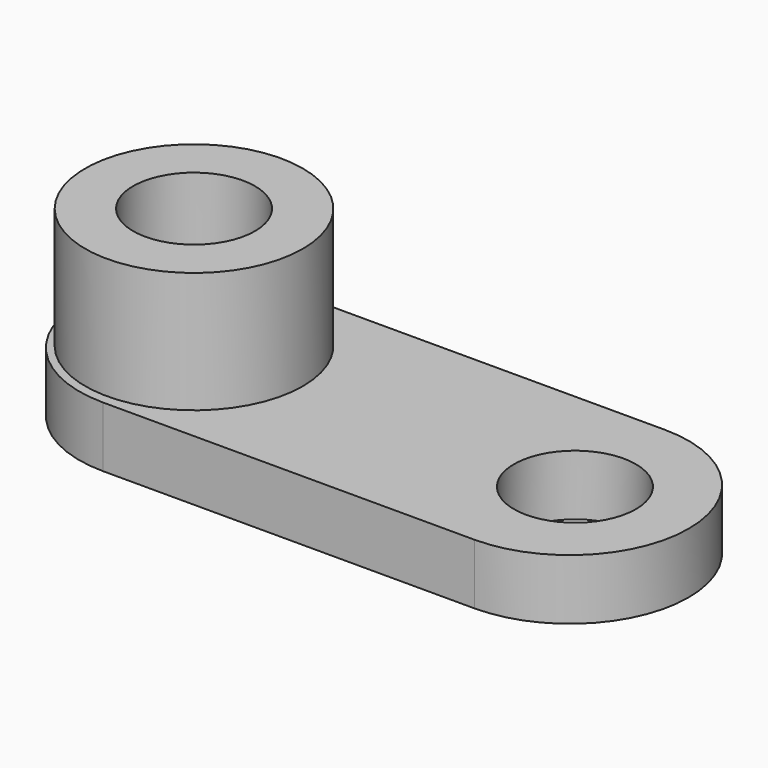
from build123d import *

# Parameters (mm, degrees)
F0_R     = 3.2
F1_DEPTH = 3.175
F2_R     = 5.715
F2_R_2   = 3.2
F3_DEPTH = 6.35


# Not quite as in the source:
# - a length typed as a fraction of an inch, garbled in the dataset ("3 / 203.2 mm" for 3/8 in), is restored


with BuildPart() as f1:
    # F0 (on Top) → F1 (new body)
    with BuildSketch(Plane.XY):
        with BuildLine():
            ThreePointArc((-5.4090924263, 50.2771637037), (-11.6590924263, 44.0271637037), (-5.4090924263, 37.7771637037))
            Line((-5.4090924263, 37.7771637037), (14.0909075737, 37.7771637037))
            ThreePointArc((14.0909075737, 37.7771637037), (20.3409075737, 44.0271637037), (14.0909075737, 50.2771637037))
            Line((14.0909075737, 50.2771637037), (-5.4090924263, 50.2771637037))
        make_face()
        with Locations((-5.6340924263, 44.0271637037)):
            Circle(F0_R, mode=Mode.SUBTRACT)
        with Locations((14.3659075737, 44.0271637037)):
            Circle(F0_R, mode=Mode.SUBTRACT)
    extrude(amount=F1_DEPTH)


with BuildPart() as f3:
    # F2 (on face) → F3 (new body)
    with BuildSketch(Plane.XY.offset(3.175)):
        with Locations((-5.6340924263, 44.0271637037)):
            Circle(F2_R)
        with Locations((-5.6340924263, 44.0271637037)):
            Circle(F2_R_2, mode=Mode.SUBTRACT)
    extrude(amount=F3_DEPTH)


solid = Compound([f1.part, f3.part])
